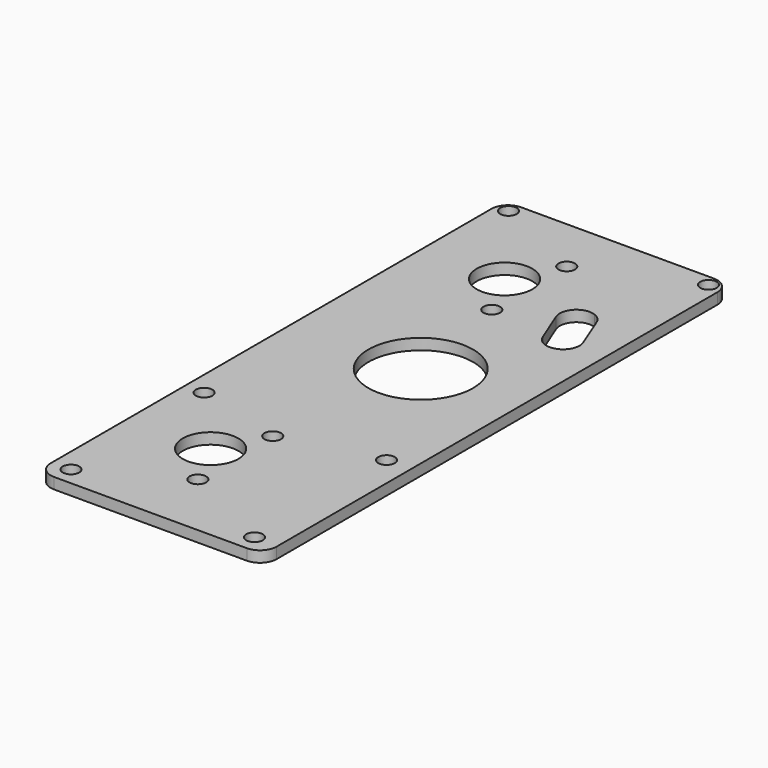
from build123d import *

# Parameters (mm, degrees)
F0_W     = 41
F0_H     = 106
F0_R     = 1.5
F0_R_2   = 5.05
F0_R_3   = 2
F0_R_4   = 9.5
F1_DEPTH = 2
F2_R     = 3


# Not quite as in the source:
# - a feature names something its author has since deleted; it is built from what else it names


with BuildPart() as f1:
    # F0 (on Top) → F1 (new body)
    with BuildSketch(Plane.XY):
        with Locations((-1.1801278293, -1.1353523731)):
            Rectangle(F0_W, F0_H)
        with Locations((-18.2301278293, -50.84027483)):
            Circle(F0_R, mode=Mode.SUBTRACT)
        with Locations((-6.776117335, -33.481924504)):
            Circle(F0_R_2, mode=Mode.SUBTRACT)
        with Locations((-18.2301278293, -20.64027483)):
            Circle(F0_R, mode=Mode.SUBTRACT)
        with Locations((-11.8353097141, -18.4490393624)):
            Circle(F0_R_3, mode=Mode.SUBTRACT)
        with BuildLine():
            ThreePointArc((0.9913514778, -28.481924504), (-4.9415118708, -25.855220261), (-8.0481067447, -20.1589485871))
            Line((-8.0481067447, -20.1589485871), (9.9913514778, -20.516399593))
            Line((9.9913514778, -20.516399593), (9.9913514778, -46.516399593))
            Line((9.9913514778, -46.516399593), (-8.0481067447, -46.804900421))
            ThreePointArc((-8.0481067447, -46.804900421), (-4.9415118708, -41.1086287471), (0.9913514778, -38.481924504))
            Line((0.9913514778, -38.481924504), (0.9913514778, -28.481924504))
        make_face(mode=Mode.SUBTRACT)
        with Locations((15.0698721707, -50.84187603)):
            Circle(F0_R, mode=Mode.SUBTRACT)
        with Locations((14.8892415527, -20.64187603)):
            Circle(F0_R, mode=Mode.SUBTRACT)
        with Locations((-11.8353097141, -0.1353523731)):
            Circle(F0_R_3, mode=Mode.SUBTRACT)
        with Locations((-11.8353097141, 18.1783346161)):
            Circle(F0_R_3, mode=Mode.SUBTRACT)
        with Locations((-19.3801278293, 49.8646476269)):
            Circle(F0_R, mode=Mode.SUBTRACT)
        with Locations((-6.776117335, 33.2112197578)):
            Circle(F0_R_2, mode=Mode.SUBTRACT)
        with Locations((1.1698721707, 4.2646476269)):
            Circle(F0_R_4, mode=Mode.SUBTRACT)
        with BuildLine():
            ThreePointArc((0.9913514778, 38.2112197578), (-4.9415118708, 40.8379240009), (-8.0481067447, 46.5341956747))
            Line((-8.0481067447, 46.5341956747), (9.9913514778, 46.2456948468))
            Line((9.9913514778, 46.2456948468), (9.9913514778, 32.6706368583))
            ThreePointArc((9.9913514778, 32.6706368583), (11.0890493373, 31.9475764467), (11.7722718766, 30.8246499525))
            Line((11.7722718766, 30.8246499525), (14.1061726006, 24.9766412934))
            ThreePointArc((14.1061726006, 24.9766412934), (14.2659629101, 24.4308184096), (14.3198721707, 23.8646476269))
            ThreePointArc((14.3198721707, 23.8646476269), (12.903292191, 21.3165540181), (9.9913514778, 21.1748460043))
            Line((9.9913514778, 21.1748460043), (9.9913514778, 20.2456948468))
            Line((9.9913514778, 20.2456948468), (-8.0481067447, 19.8882438409))
            ThreePointArc((-8.0481067447, 19.8882438409), (-4.9415118708, 25.5845155147), (0.9913514778, 28.2112197578))
            Line((0.9913514778, 28.2112197578), (0.9913514778, 38.2112197578))
        make_face(mode=Mode.SUBTRACT)
        with Locations((16.9198721707, 49.8646476269)):
            Circle(F0_R, mode=Mode.SUBTRACT)
        with BuildLine():
            Line((9.9913514778, -20.516399593), (-8.0481067447, -20.1589485871))
            ThreePointArc((-8.0481067447, -20.1589485871), (-4.9415118708, -25.855220261), (0.9913514778, -28.481924504))
            Line((0.9913514778, -28.481924504), (0.9913514778, -38.481924504))
            ThreePointArc((0.9913514778, -38.481924504), (-4.9415118708, -41.1086287471), (-8.0481067447, -46.804900421))
            Line((-8.0481067447, -46.804900421), (9.9913514778, -46.516399593))
            Line((9.9913514778, -46.516399593), (9.9913514778, -20.516399593))
        make_face()
        with Locations((-2.2937730764, -41.981924504)):
            Circle(F0_R, mode=Mode.SUBTRACT)
        with Locations((-2.2937730764, -24.981924504)):
            Circle(F0_R, mode=Mode.SUBTRACT)
        with BuildLine():
            Line((9.9913514778, 46.2456948468), (-8.0481067447, 46.5341956747))
            ThreePointArc((-8.0481067447, 46.5341956747), (-4.9415118708, 40.8379240009), (0.9913514778, 38.2112197578))
            Line((0.9913514778, 38.2112197578), (0.9913514778, 28.2112197578))
            ThreePointArc((0.9913514778, 28.2112197578), (-4.9415118708, 25.5845155147), (-8.0481067447, 19.8882438409))
            Line((-8.0481067447, 19.8882438409), (9.9913514778, 20.2456948468))
            Line((9.9913514778, 20.2456948468), (9.9913514778, 21.1748460043))
            ThreePointArc((9.9913514778, 21.1748460043), (9.1863324168, 21.7556174899), (8.614900686, 22.5672929078))
            ThreePointArc((8.614900686, 22.5672929078), (8.5339821319, 22.7516262021), (8.4656083094, 22.9409713794))
            Line((8.4656083094, 22.9409713794), (6.1441299956, 28.7516262021))
            ThreePointArc((6.1441299956, 28.7516262021), (6.7891821801, 31.9662692108), (9.9913514778, 32.6706368583))
            Line((9.9913514778, 32.6706368583), (9.9913514778, 46.2456948468))
        make_face()
        with Locations((-2.2937730764, 24.7112197578)):
            Circle(F0_R, mode=Mode.SUBTRACT)
        with Locations((-2.2937730764, 41.7112197578)):
            Circle(F0_R, mode=Mode.SUBTRACT)
        with Locations((-11.8353097141, -18.4490393624)):
            Circle(F0_R_3)
        with Locations((-11.8353097141, -0.1353523731)):
            Circle(F0_R_3)
        with Locations((-11.8353097141, 18.1783346161)):
            Circle(F0_R_3)
    extrude(amount=F1_DEPTH)

    # F2
    f2_edges = [f1.edges().sort_by_distance(p)[0] for p in [
        (-21.680128, 51.864648, 1),
        (-21.680128, -54.135352, 1),
        (19.319872, -54.135352, 1),
        (19.319872, 51.864648, 1),
    ]]
    fillet(f2_edges, radius=F2_R)


solid = f1.part
